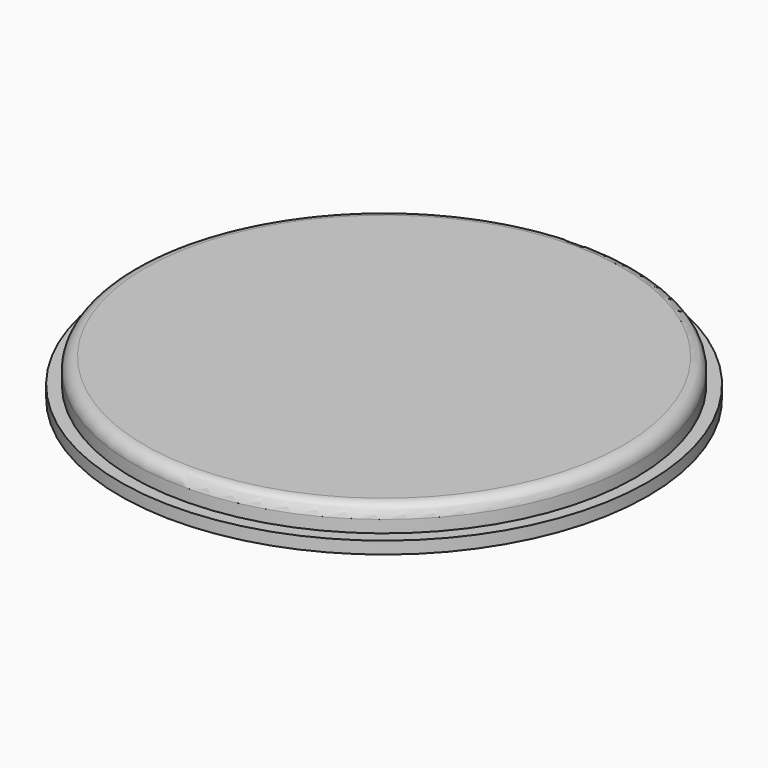
from build123d import *

# Parameters (mm, degrees)
F0_R     = 107.5
F1_DEPTH = 5
F2_R     = 100
F3_DEPTH = 6
F4_R     = 102.5
F4_R_2   = 100
F5_DEPTH = 5
F6_R     = 102.5
F7_DEPTH = 5
F8_R     = 4.99999


# Not quite as in the source:
# - a fillet or chamfer is up to 0.001 mm smaller than in the source, because OpenCascade refuses the exact size


with BuildPart() as f1:
    # F0 (on Top) → F1 (new body)
    with BuildSketch(Plane.XY):
        Circle(F0_R)
    extrude(amount=F1_DEPTH)

    # F2 (on face) → F3 (cut)
    with BuildSketch(Plane.XY.offset(5)):
        Circle(F2_R)
    extrude(amount=-F3_DEPTH, mode=Mode.SUBTRACT)

    # F4 (on face) → F5 (join)
    with BuildSketch(Plane.XY.offset(5)):
        Circle(F4_R)
        Circle(F4_R_2, mode=Mode.SUBTRACT)
    extrude(amount=F5_DEPTH)

    # F6 (on face) → F7 (join)
    with BuildSketch(Plane.XY.offset(10)):
        Circle(F6_R)
    extrude(amount=F7_DEPTH)

    # F8 (radius 5 in the source; OpenCascade refuses exactly that, so slightly less here)
    f8_edges = [f1.edges().sort_by_distance(p)[0] for p in [
        (-102.5, 0, 15),
    ]]
    fillet(f8_edges, radius=F8_R)


solid = f1.part
